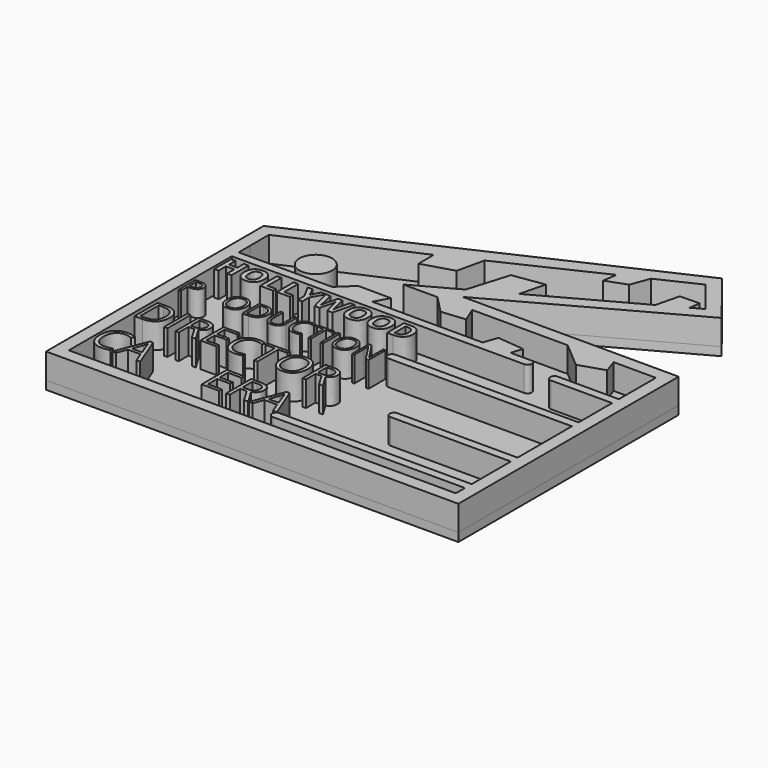
from build123d import *

# Parameters (mm, degrees)
F0_R           = 3.8941334831
F0_TEXT_SIZE   = 10.4319842225
F0_TEXT_SIZE_2 = 6.9875633215
F0_TEXT_SIZE_3 = 9.6164666511
F0_TEXT_SIZE_4 = 7.0313704153
F1_DEPTH       = 6
F3_DEPTH       = 2


# Not quite as in the source:
# - Text() gives the source's letters only with a copy of the font that has no kerning and outlines rounded to 1/6400 em; it was checked with that copy


with BuildPart() as f1:
    # F0 (on Top) → F1 (new body)
    with BuildSketch(Plane.XY):
        Polygon((-49.2642200291, -11.3319797484), (-49.2642200291, -16.9781416899), (-49.2642200291, -54.3686768084), (-49.2642200291, -56.6767749959), (-46.2174160705, -56.6767749959), (45.1263809228, -56.6767749959), (48.5641956329, -56.6767749959), (48.5641956329, 8.6092837155), (48.5641956329, 8.657189184), (-2.6406015009, 8.657189184), (40.0808416307, 32.0296697319), (30.2105510753, 44.4407714677), (-49.2642200291, 7.8356554749), (-49.2642200291, 5.5755445682), (-49.2642200291, 0), align=None)
        with BuildLine():
            Line((-14.3747102727, 5.657189184), (-11.3800320792, 5.657189184))
            Line((-11.3800320792, 5.657189184), (-6.256897775, 5.657189184))
            Line((-6.256897775, 5.657189184), (-2.1628705101, 1.4384416149))
            Line((-2.1628705101, 1.4384416149), (3.4810829802, 1.9917704185))
            Line((3.4810829802, 1.9917704185), (1.9769035375, 5.657189184))
            Line((1.9769035375, 5.657189184), (24.6255436904, 5.657189184))
            Line((24.6255436904, 5.657189184), (30.7268623553, 0.4913766886))
            Line((30.7268623553, 0.4913766886), (36.6205491416, 2.3818044708))
            Line((36.6205491416, 2.3818044708), (35.5524160797, 5.657189184))
            Line((35.5524160797, 5.657189184), (45.5641956329, 5.657189184))
            Line((45.5641956329, 5.657189184), (45.5641956329, -5.3273318335))
            Line((45.5641956329, -5.3273318335), (31.0842806631, -5.3273318335))
            ThreePointArc((31.0842806631, -5.3273318335), (30.0842806631, -6.3273318335), (31.0842806631, -7.3273318335))
            Line((31.0842806631, -7.3273318335), (45.5641956329, -7.3273318335))
            Line((45.5641956329, -7.3273318335), (45.5641956329, -17.2513987422))
            Line((45.5641956329, -17.2513987422), (2.0775083582, -17.2513987422))
            ThreePointArc((2.0775083582, -17.2513987422), (1.0775083582, -18.2513987422), (2.0775083582, -19.2513987422))
            Line((2.0775083582, -19.2513987422), (45.5641956329, -19.2513987422))
            Line((45.5641956329, -19.2513987422), (45.5641956329, -35.3619152752))
            Line((45.5641956329, -35.3619152752), (17.0290430559, -35.3619152752))
            ThreePointArc((17.0290430559, -35.3619152752), (16.0290430559, -36.3619152752), (17.0290430559, -37.3619152752))
            Line((17.0290430559, -37.3619152752), (45.5641956329, -37.3619152752))
            Line((45.5641956329, -37.3619152752), (45.5641956329, -48.9762909867))
            Line((45.5641956329, -48.9762909867), (0, -48.9762909867))
            ThreePointArc((0, -48.9762909867), (-1, -49.9762909867), (0, -50.9762909867))
            Line((0, -50.9762909867), (45.5641956329, -50.9762909867))
            Line((45.5641956329, -50.9762909867), (45.5641956329, -53.6767749959))
            Line((45.5641956329, -53.6767749959), (-46.2642200291, -53.6767749959))
            Line((-46.2642200291, -53.6767749959), (-46.2642200291, -28.4380592864))
            Line((-46.2642200291, -28.4380592864), (-46.2642200291, -22.0373139562))
            Line((-46.2642200291, -22.0373139562), (-46.2642200291, -16.9747272572))
            Line((-46.2642200291, -16.9747272572), (-46.2642200291, -11.3336763284))
            Line((-46.2642200291, -11.3336763284), (-46.2642200291, -5.3273318335))
            Line((-46.2642200291, -5.3273318335), (23.1031794046, -5.3273318335))
            ThreePointArc((23.1031794046, -5.3273318335), (24.1031794046, -4.3273318335), (23.1031794046, -3.3273318335))
            Line((23.1031794046, -3.3273318335), (18.3010469499, -3.3273318335))
            Line((18.3010469499, -3.3273318335), (19.1029366106, -0.6601023488))
            Line((19.1029366106, -0.6601023488), (12.7742873264, -0.0545488606))
            Line((12.7742873264, -0.0545488606), (11.636915419, -3.3273318335))
            Line((11.636915419, -3.3273318335), (-14.5309058367, -3.3273318335))
            Line((-14.5309058367, -3.3273318335), (-12.7649698406, -0.0548266144))
            Line((-12.7649698406, -0.0548266144), (-20.5262228847, 0))
            Line((-20.5262228847, 0), (-24.0490497772, -3.3273318335))
            Line((-24.0490497772, -3.3273318335), (-46.2174160705, -3.3273318335))
            Line((-46.2174160705, -3.3273318335), (-46.2642200291, 0))
            Line((-46.2642200291, 0), (-46.2642200291, 5.657189184))
            Line((-46.2642200291, 5.657189184), (-17.3906497657, 18.4475872666))
            Line((-17.3906497657, 18.4475872666), (-17.3856895839, 18.449935489))
            Line((-17.3856895839, 18.449935489), (-17.3856895839, 13.9446656039))
            Line((-17.3856895839, 13.9446656039), (-10.0837424819, 16.1290091282))
            Line((-10.0837424819, 16.1290091282), (-8.6255447404, 22.5971157783))
            Line((-8.6255447404, 22.5971157783), (14.0760365063, 33.3443753231))
            Line((14.0760365063, 33.3443753231), (13.5637551295, 30.007432201))
            Line((13.5637551295, 30.007432201), (18.3647835376, 31.7532596971))
            Line((18.3647835376, 31.7532596971), (20.0104204638, 36.1537992103))
            Line((20.0104204638, 36.1537992103), (29.4238416816, 40.6102500598))
            Line((29.4238416816, 40.6102500598), (35.5148598579, 32.9512813762))
            Line((35.5148598579, 32.9512813762), (32.88562743, 31.5128542241))
            Line((32.88562743, 31.5128542241), (33.2495834205, 34.0587258442))
            Line((33.2495834205, 34.0587258442), (28.5916565199, 33.9591970392))
            Line((28.5916565199, 33.9591970392), (27.2312564416, 28.4194035762))
            Line((27.2312564416, 28.4194035762), (4.7506091163, 16.1204629553))
            Line((4.7506091163, 16.1204629553), (6.2568720721, 22.1349620977))
            Line((6.2568720721, 22.1349620977), (-1.1445954617, 21.0415558674))
            Line((-1.1445954617, 21.0415558674), (-4.0805555051, 11.2890198158))
            Line((-4.0805555051, 11.2890198158), (-14.3747102727, 5.657189184))
        make_face(mode=Mode.SUBTRACT)
        with Locations((-32.0606976748, 1.8139833119)):
            Circle(F0_R)
        with Locations((-46.2642200291, -48.9762909867)):
            Text('CA     ERA', F0_TEXT_SIZE, font='Open Sans', text_align=(TextAlign.LEFT, TextAlign.BOTTOM))
        with Locations((-46.2642200291, -11.3336763284)):
            Text('HOLLYWOOD', F0_TEXT_SIZE_2, font='Open Sans', font_style=FontStyle.BOLD, text_align=(TextAlign.LEFT, TextAlign.BOTTOM))
        with Locations((-46.2642200291, -35.3619152752)):
            Text('DIRECTOR', F0_TEXT_SIZE_3, font='Open Sans', text_align=(TextAlign.LEFT, TextAlign.BOTTOM))
        with Locations((-46.2642200291, -22.0373139562)):
            Text('P   ODUCTION', F0_TEXT_SIZE_4, font='Open Sans', text_align=(TextAlign.LEFT, TextAlign.BOTTOM))
    extrude(amount=F1_DEPTH)


with BuildPart() as f3:
    # F2 (on Top) → F3 (new body)
    with BuildSketch(Plane.XY):
        Polygon((48.5641956329, 8.657189184), (-2.6406015009, 8.657189184), (40.0808416307, 32.0296697319), (30.2105510753, 44.4407714677), (-49.2642200291, 7.8356554749), (-49.2642200291, -56.6767749959), (48.5641956329, -56.6767749959), align=None)
    extrude(amount=-F3_DEPTH)


solid = Compound([f1.part, f3.part])
